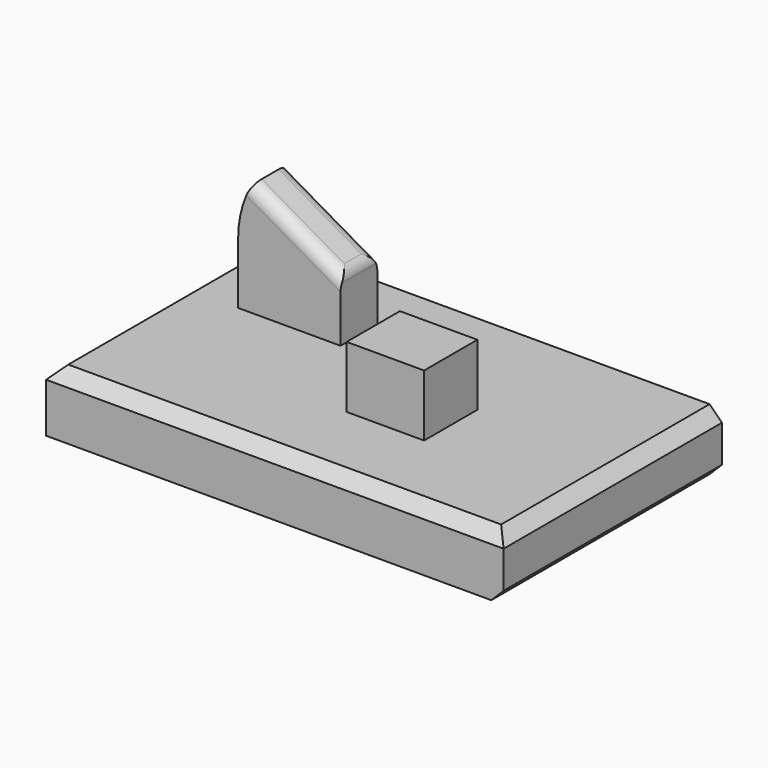
from build123d import *

# Parameters (mm, degrees)
F0_W      = 185.4944750667
F0_H      = 110.638756305
F1_DEPTH  = 25
F2_SIZE   = 5
F3_W      = 31.4006619155
F3_H      = 26.9978269935
F3_W_2    = 41.5280163288
F3_H_2    = 18.5919255018
F4_DEPTH  = 25
F4_FACE_W = 41.5280163288
F4_FACE_H = 18.5919255018
F5_ANGLE  = 30
F6_R      = 5


with BuildPart() as f1:
    # F0 (on Top) → F1 (new body)
    with BuildSketch(Plane.XY):
        with Locations((57.9323507845, 20.6255745143)):
            Rectangle(F0_W, F0_H)
    extrude(amount=F1_DEPTH)

    # F2
    f2_edges = [f1.edges().sort_by_distance(p)[0] for p in [
        (57.932351, -34.693804, 25),
        (-34.814887, 20.625575, 25),
        (150.679588, 20.625575, 25),
        (150.679588, 20.625575, 0),
    ]]
    chamfer(f2_edges, length=F2_SIZE)

    # F3 (on face) → F4 (join)
    with BuildSketch(Plane.XY.offset(25)):
        with Locations((74.988739565, 13.4989134967)):
            Rectangle(F3_W, F3_H)
        with Locations((8.6979772896, 43.5124337673)):
            Rectangle(F3_W_2, F3_H_2)
    extrude(amount=F4_DEPTH)

    # F4_face (on face) → F5 (revolve)
    with BuildSketch(Plane(origin=(8.6979772896, 43.5124337673, 50), x_dir=(1, 0, 0), z_dir=(0, 0, 1))):
        Rectangle(F4_FACE_W, F4_FACE_H)
    revolve(axis=Axis((29.461985454, 43.5124337673, 50), (0, 1, 0)), revolution_arc=F5_ANGLE)

    # F6
    f6_edges = [f1.edges().sort_by_distance(p)[0] for p in [
        (11.479827, 34.216471, 60.382004),
        (11.479827, 52.808397, 60.382004),
        (29.461985, 43.512434, 50),
    ]]
    fillet(f6_edges, radius=F6_R)


solid = f1.part
